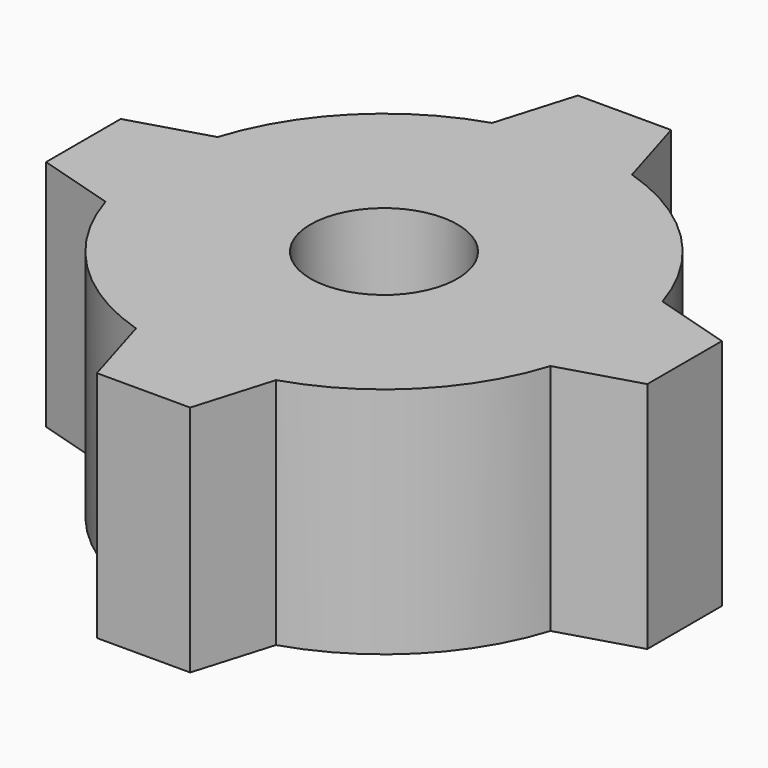
from build123d import *

# Parameters (mm, degrees)
F1_DEPTH = 10
F3_DEPTH = 4
F4_D     = 6.3
F5_DEPTH = 10
F7_COUNT = 4


with BuildPart() as f1:
    # F0 (on Top) → F1 (new body)
    with BuildSketch(Plane.XY):
        with BuildLine():
            ThreePointArc((3, -9.5393920142), (8.0622577483, -5.9160797831), (10, 0))
            ThreePointArc((10, 0), (-5.9160797831, 8.0622577483), (-3, -9.5393920142))
            ThreePointArc((-3, -9.5393920142), (0, -10), (3, -9.5393920142))
        make_face()
    extrude(amount=F1_DEPTH)

    # F2 (on face) → F3 (cut)
    with BuildSketch(Plane(origin=(0, 0, 0), x_dir=(1, 0, 0), z_dir=(0, 0, -1))):
        Polygon((-2.8867513459, -5), (2.8867513459, -5), (5.7735026919, 0), (2.8867513459, 5), (-2.8867513459, 5), (-5.7735026919, 0), align=None)
    extrude(amount=-F3_DEPTH, mode=Mode.SUBTRACT)

    # F4 (through all)
    with Locations(Plane(origin=(0, 0, 0), x_dir=(1, 0, 0), z_dir=(0, 0, -1))):
        with Locations((0, 0)):
            Hole(F4_D / 2)



with BuildPart() as f5:
    # F0 (on Top) → F5 (new body, through all)
    with BuildSketch(Plane.XY):
        with BuildLine():
            ThreePointArc((3, -9.5393920142), (0, -10), (-3, -9.5393920142))
            Line((-3, -9.5393920142), (-2, -12.8883451594))
            Line((-2, -12.8883451594), (0, -12.8883451594))
            Line((0, -12.8883451594), (2, -12.8883451594))
            Line((2, -12.8883451594), (3, -9.5393920142))
        make_face()
    extrude(amount=F5_DEPTH)


with BuildPart() as f1_1:
    add(f1.part)

    add(f5.part)  # F7 merges F5
    # F7: F5 ×4 about axis
    f7_axis = Axis((0, 0, -12.0245739818), (0, 0, -1))
    for i in range(1, F7_COUNT):
        add(f5.part.rotate(f7_axis, i * 360 / F7_COUNT))


solid = f1_1.part
